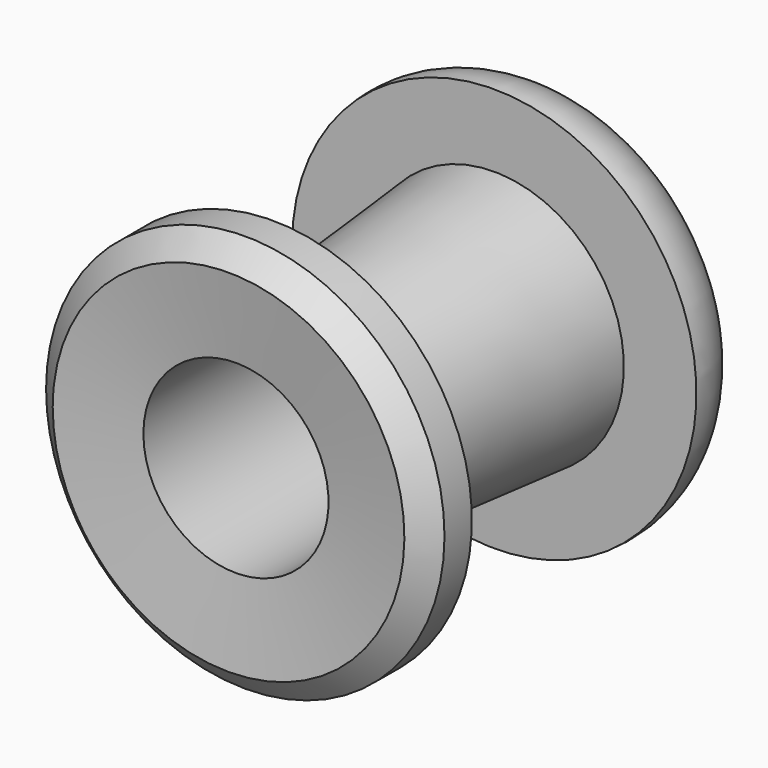
from build123d import *

# Parameters (mm, degrees)
F3_SIZE  = 5.08
F5_DEPTH = 25.4


# Not quite as in the source:
# - a fillet or chamfer that OpenCascade refuses, or shapes differently, is made with other operations: its cross-section is extruded or revolved along the edge and cut away or added


with BuildPart() as f1:
    # F0 (on Top) → F1 (revolve)
    with BuildSketch(Plane.XY):
        Polygon((-19.9900865555, -40.7797805965), (-19.9900865555, 45.5773994327), (-51.6543835402, 45.5773994327), (-43.658349663, 28.9456453174), (-27.9861204326, 28.9456453174), (-23.8281842321, -19.3504039198), (-43.0186651647, -30.8646950871), (-43.0186651647, -43.3385074139), align=None)
    revolve(axis=Axis((0, -1.2793652713, 0), (0, -1, 0)))

    # F2: fillet of radius 15.0328655844 on 1 edges, made by hand

    # F2_s1 → F2_t2 (revolve, cut)
    with BuildSketch(Plane.XY):
        with BuildLine():
            ThreePointArc((-28.7107544335, 45.5773994327), (-39.8916069066, 40.5931947369), (-43.658349663, 28.9456453174))
            Line((-43.658349663, 28.9456453174), (-51.6543835402, 45.5773994327))
            Line((-51.6543835402, 45.5773994327), (-28.7107544335, 45.5773994327))
        make_face()
    revolve(axis=Axis((0, 45.5773994327, 0), (0, -1, 0)), mode=Mode.SUBTRACT)

    # F3
    f3_edges = [f1.edges().sort_by_distance(p)[0] for p in [
        (43.018665, -43.338507, 0),
    ]]
    chamfer(f3_edges, length=F3_SIZE)

    # F4 (on face) → F5 (join)
    with BuildSketch(Plane(origin=(0, 45.5773994327, 0), x_dir=(-1, 0, 0), z_dir=(0, 1, 0))):
        with BuildLine():
            ThreePointArc((1.7598816693, -28.6567659838), (12.6790964927, -25.7594241448), (21.635263345, -18.8738655324))
            ThreePointArc((21.635263345, -18.8738655324), (18.1448647045, -15.8726036273), (13.7469387774, -14.5129333612))
            ThreePointArc((13.7469387774, -14.5129333612), (8.8279197581, -17.9351998383), (3.1156176835, -19.7457966906))
            ThreePointArc((3.1156176835, -19.7457966906), (1.5105456445, -24.0602143155), (1.7598816693, -28.6567659838))
        make_face()
    extrude(amount=F5_DEPTH)


solid = f1.part
